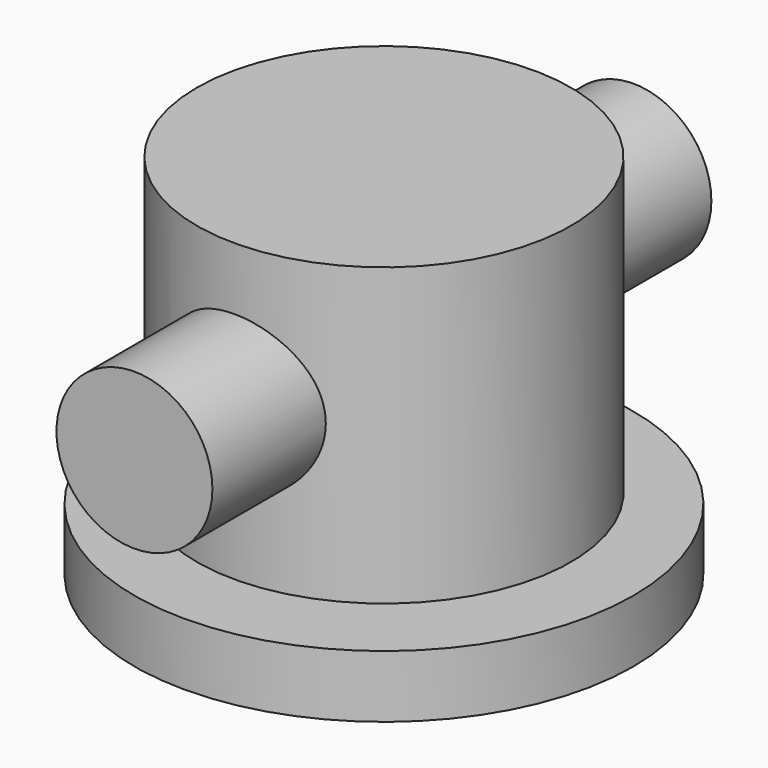
from build123d import *

# Parameters (mm, degrees)
F2_R      = 1
F3_DEPTH  = 4
F4_R      = 0.5
F7_R      = 2.5
F8_DEPTH  = 10
F11_W     = 3
F11_H     = 10
F12_DEPTH = 8.2


with BuildPart() as f1:
    # F0 (on Front) → F1 (revolve)
    with BuildSketch(Plane.XZ):
        Polygon((0, 0), (0, 8), (-3.5, 8), (-3.5, 0), (-8, 0), (-8, -2), (0, -2), align=None)
    revolve(axis=Axis((0, 0, 4), (0, 0, 1)))

    # F2 (on Front) → F3 (join, symmetric)
    with BuildSketch(Plane.XZ):
        with Locations((0, 7)):
            Circle(F2_R)
    extrude(amount=F3_DEPTH, both=True)

    # F4
    f4_edges = [f1.edges().sort_by_distance(p)[0] for p in [
        (-1, -4, 7),
        (-1, 4, 7),
    ]]
    fillet(f4_edges, radius=F4_R)


with BuildPart() as f6:
    # F5 (on Front) → F6 (revolve)
    with BuildSketch(Plane.XZ):
        Polygon((-3.7, 0.3), (-3.7, 8.2), (0, 8.2), (0, 9.7907921299), (-6, 9.7907921299), (-6, 0.3), align=None)
    revolve(axis=Axis((0, 0, 8.995396065), (0, 0, 1)))

    # F7 (on Front) → F8 (join, symmetric)
    with BuildSketch(Plane.XZ):
        with Locations((0, 5.2907921299)):
            Circle(F7_R)
    extrude(amount=F8_DEPTH, both=True)

    # F9 (on Front) → F10 (revolve, cut)
    with BuildSketch(Plane.XZ):
        Polygon((0, 0.3), (0, 8.2), (-3.7, 8.2), (-5, 8.2), (-5, 5.6), (-3.7, 5.6), (-3.7, 0.3), align=None)
    revolve(axis=Axis((0, 0, 4.25), (0, 0, -1)), mode=Mode.SUBTRACT)

    # F11 (on Top) → F12 (cut, through all)
    with BuildSketch(Plane.XY):
        Rectangle(F11_W, F11_H)
    extrude(amount=F12_DEPTH, mode=Mode.SUBTRACT)


solid = Compound([f1.part, f6.part])
